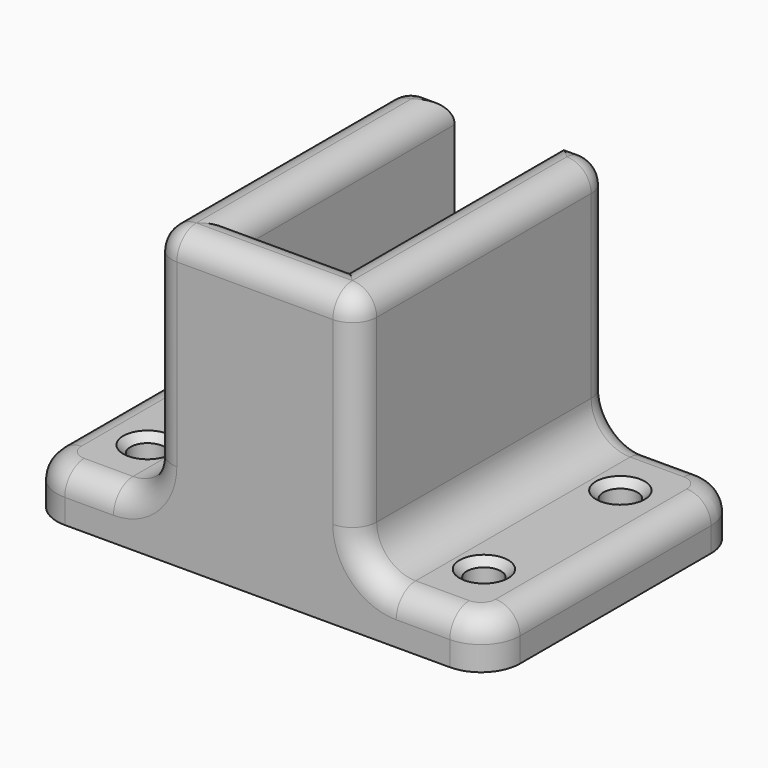
from build123d import *

# Parameters (mm, degrees)
F0_W           = 95
F0_H           = 65
F1_DEPTH       = 10
F3_DEPTH       = 50
F4_R           = 8
F5_R           = 4.99999
F7_D           = 7
F7_CSINK_D     = 10
F7_CSINK_ANGLE = 90
F8_T1_DEPTH    = 30
F8_T4_ANGLE    = 90
F8_T6_ANGLE    = 90
F8_T8_ANGLE    = 90
F8_T10_ANGLE   = 90


# Not quite as in the source:
# - a fillet or chamfer that OpenCascade refuses, or shapes differently, is made with other operations: its cross-section is extruded or revolved along the edge and cut away or added
# - a fillet or chamfer is up to 0.001 mm smaller than in the source, because OpenCascade refuses the exact size


with BuildPart() as f1:
    # F0 (on Top) → F1 (new body)
    with BuildSketch(Plane.XY):
        with Locations((47.5, 32.5)):
            Rectangle(F0_W, F0_H)
    extrude(amount=F1_DEPTH)

    # F2 (on face) → F3 (join)
    with BuildSketch(Plane.XY.offset(10)):
        Polygon((36, 65), (26, 65), (26, 0), (68, 0), (68, 65), (58, 65), (58, 10), (36, 10), align=None)
    extrude(amount=F3_DEPTH)

    # F4
    f4_edges = [f1.edges().sort_by_distance(p)[0] for p in [
        (68, 32.5, 10),
        (26, 32.5, 10),
    ]]
    fillet(f4_edges, radius=F4_R)

    # F5 (radius 5 in the source; OpenCascade refuses exactly that, so slightly less here)
    f5_edges = [f1.edges().sort_by_distance(p)[0] for p in [
        (85.5, 65, 10),
        (76, 32.5, 10),
        (95, 32.5, 10),
        (85.5, 0, 10),
        (9, 65, 10),
        (18, 32.5, 10),
        (0, 32.5, 10),
        (9, 0, 10),
        (31, 65, 60),
        (26, 32.5, 60),
        (47, 0, 60),
        (68, 32.5, 60),
        (63, 65, 60),
        (58, 37.5, 60),
        (47, 10, 60),
        (36, 37.5, 60),
    ]]
    fillet(f5_edges, radius=F5_R)

    # F7 (through all)
    with Locations(Plane.XY.offset(10)):
        with Locations((13, 50), (13, 15), (82, 50), (82, 15)):
            CounterSinkHole(F7_D / 2, F7_CSINK_D / 2, counter_sink_angle=F7_CSINK_ANGLE)

    # F8: fillet of radius 8 on 4 edges, made by hand

    # F8_s2 → F8_t1 (cut)
    with BuildSketch(Plane.XY.offset(-20)):
        with BuildLine():
            ThreePointArc((8, 65), (2.3431457505, 62.6568542495), (0, 57))
            Line((0, 57), (0, 65))
            Line((0, 65), (8, 65))
        make_face()
        with BuildLine():
            ThreePointArc((87, 65), (92.6568542495, 62.6568542495), (95, 57))
            Line((95, 57), (95, 65))
            Line((95, 65), (87, 65))
        make_face()
        with BuildLine():
            ThreePointArc((95, 8), (92.6568542495, 2.3431457505), (87, 0))
            Line((87, 0), (95, 0))
            Line((95, 0), (95, 8))
        make_face()
        with BuildLine():
            ThreePointArc((0, 8), (2.3431457505, 2.3431457505), (8, 0))
            Line((8, 0), (0, 0))
            Line((0, 0), (0, 8))
        make_face()
    extrude(amount=F8_T1_DEPTH, mode=Mode.SUBTRACT)

    # F8_s3 → F8_t4 (revolve, cut)
    with BuildSketch(Plane.XZ.offset(-8)):
        with BuildLine():
            ThreePointArc((4.99999, 10), (1.4644631651, 8.5355368349), (0, 5.00001))
            Line((0, 5.00001), (0, 10))
            Line((0, 10), (4.99999, 10))
        make_face()
    revolve(axis=Axis((8, 8, 10), (0, 0, 1)), revolution_arc=F8_T4_ANGLE, mode=Mode.SUBTRACT)

    # F8_s5 → F8_t6 (revolve, cut)
    with BuildSketch(Plane.YZ.offset(87)):
        with BuildLine():
            ThreePointArc((4.99999, 10), (1.4644631651, 8.5355368349), (0, 5.00001))
            Line((0, 5.00001), (0, 10))
            Line((0, 10), (4.99999, 10))
        make_face()
    revolve(axis=Axis((87, 8, 10), (0, 0, 1)), revolution_arc=F8_T6_ANGLE, mode=Mode.SUBTRACT)

    # F8_s7 → F8_t8 (revolve, cut)
    with BuildSketch(Plane.XZ.offset(-57)):
        with BuildLine():
            ThreePointArc((90.00001, 10), (93.5355368349, 8.5355368349), (95, 5.00001))
            Line((95, 5.00001), (95, 10))
            Line((95, 10), (90.00001, 10))
        make_face()
    revolve(axis=Axis((87, 57, 10), (0, 0, 1)), revolution_arc=F8_T8_ANGLE, mode=Mode.SUBTRACT)

    # F8_s9 → F8_t10 (revolve, cut)
    with BuildSketch(Plane.YZ.offset(8)):
        with BuildLine():
            ThreePointArc((60.00001, 10), (63.5355368349, 8.5355368349), (65, 5.00001))
            Line((65, 5.00001), (65, 10))
            Line((65, 10), (60.00001, 10))
        make_face()
    revolve(axis=Axis((8, 57, 10), (0, 0, 1)), revolution_arc=F8_T10_ANGLE, mode=Mode.SUBTRACT)


solid = f1.part
